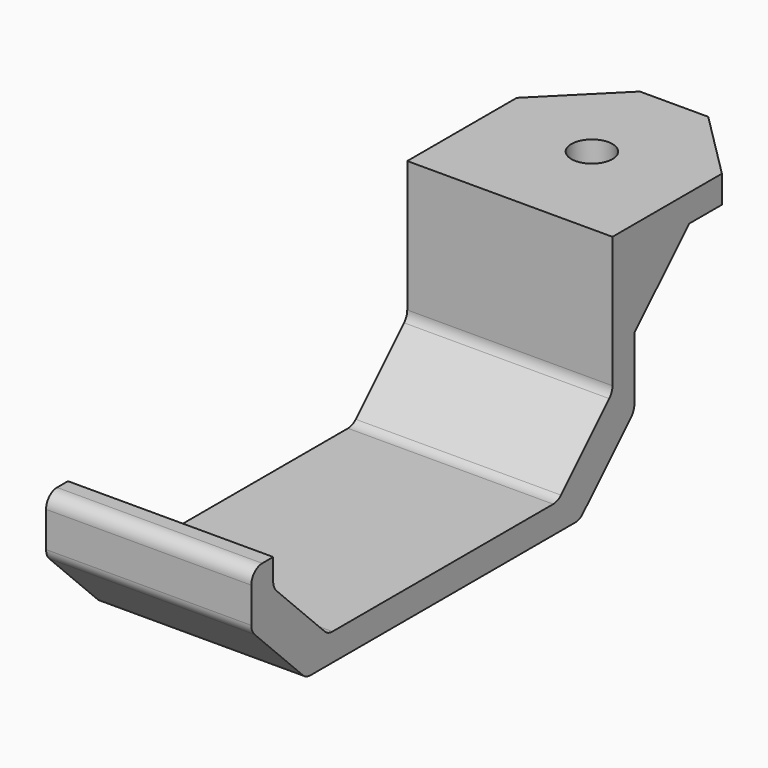
from build123d import *

# Parameters (mm, degrees)
F1_DEPTH       = 15
F2_DEPTH       = 2
F4_D           = 3
F4_DEPTH       = 100
F4_CBORE_D     = 10
F4_CBORE_DEPTH = 0.2
F4_TIP         = 0.9012909285
F5_T1_DEPTH    = 15
F5_T6_DEPTH    = 13
F5_S7_R        = 5
F5_T8_DEPTH    = 9
F5_T9_DEPTH    = 40.7168298797
F5_T11_DEPTH   = 27.7168298797
F6_R           = 1


# Not quite as in the source:
# - a fillet or chamfer that OpenCascade refuses, or shapes differently, is made with other operations: its cross-section is extruded or revolved along the edge and cut away or added


with BuildPart() as f1:
    # F0 (on Right) → F1 (new body)
    with BuildSketch(Plane.YZ):
        Polygon((-35, 9), (-35, 0), (0, 0), (0, 7.5), (0, 15), (6.5, 15), (13, 15), (13, 17), (-2, 17), (-2, 2), (-33, 2), (-33, 9), align=None)
    extrude(amount=F1_DEPTH)

    # F0 (on Right) → F2 (join)
    with BuildSketch(Plane.YZ):
        Polygon((0, 15), (0, 7.5), (6.5, 15), align=None)
    extrude(amount=F2_DEPTH)

    # F4
    with Locations(Plane(origin=(0, 0, 15), x_dir=(1, 0, 0), z_dir=(0, 0, -1))):
        with Locations((7.5, -5.5)):
            CounterBoreHole(F4_D / 2, F4_CBORE_D / 2, F4_CBORE_DEPTH, depth=F4_DEPTH)
            with Locations((0, 0, -(F4_DEPTH + F4_TIP / 2))):  # 118° drill point
                Cone(0, F4_D / 2, F4_TIP, mode=Mode.SUBTRACT)

    # F5: chamfer of 5 on 7 edges, made by hand

    # F5_s2 → F5_t1 (join)
    with BuildSketch(Plane.YZ):
        Polygon((-2, 7), (-7, 2), (-2, 2), align=None)
        Polygon((-33, 7), (-28, 2), (-33, 2), align=None)
    extrude(amount=F5_T1_DEPTH)


with BuildPart() as f5_tool4:
    # F5_s5 → F5_t6 (new body)
    with BuildSketch(Plane.YZ.offset(2)):
        Polygon((0, 10), (5, 15), (0, 15), align=None)
    extrude(amount=F5_T6_DEPTH)

    # F5_s7 → F5_t8 (cut, symmetric)
    with BuildSketch(Plane.XY.offset(12.5)):
        with Locations((7.5, 5.5)):
            Circle(F5_S7_R)
    extrude(amount=F5_T8_DEPTH, both=True, mode=Mode.SUBTRACT)


with BuildPart() as f1_1:
    add(f1.part)

    # F5_t3: union F5_tool4
    add(f5_tool4.part)

    # F5_s10 → F5_t9 (cut)
    with BuildSketch(Plane.YZ.offset(-12.8584149398)):
        Polygon((-35, 5), (-30, 0), (-35, 0), align=None)
        Polygon((-5, 0), (0, 5), (0, 0), align=None)
    extrude(amount=F5_T9_DEPTH, mode=Mode.SUBTRACT)

    # F5_s12 → F5_t11 (cut)
    with BuildSketch(Plane.XY.offset(2.1415850602)):
        Polygon((15, 8), (10, 13), (15, 13), align=None)
        Polygon((0, 8), (5, 13), (0, 13), align=None)
    extrude(amount=F5_T11_DEPTH, mode=Mode.SUBTRACT)

    # F6
    f6_edges = [f1_1.edges().sort_by_distance(p)[0] for p in [
        (7.5, -35, 9),
        (7.5, 0, 5),
        (7.5, -5, 0),
        (7.5, -30, 0),
        (7.5, -35, 5),
        (7.5, -33, 7),
        (7.5, -28, 2),
        (7.5, -7, 2),
        (7.5, -2, 7),
    ]]
    fillet(f6_edges, radius=F6_R)


solid = f1_1.part
